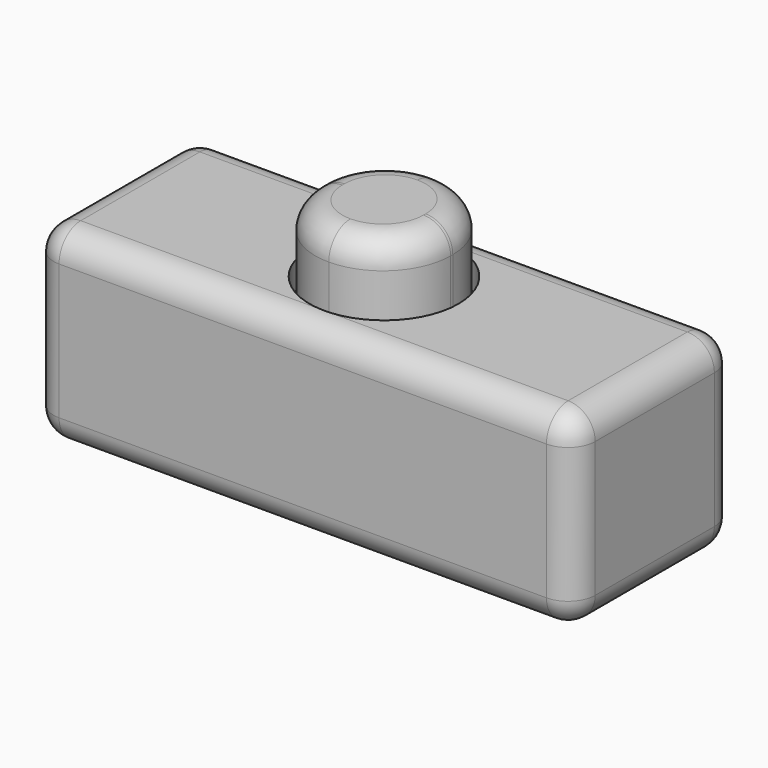
from build123d import *

# Parameters (mm, degrees)
F0_W     = 50.8
F0_H     = 19.05
F0_W_2   = 45.72
F0_H_2   = 13.97
F1_DEPTH = 12.7
F2_W     = 50.8
F2_H     = 19.05
F3_DEPTH = 2.54
F5_START = 0.508
F4_W     = 4.572
F4_H     = 2.794
F4_W_2   = 12.7
F4_H_2   = 5.08
F4_H_3   = 3.81
F5_DEPTH = 12.954
F6_R     = 6.34999
F7_W     = 50.8
F7_H     = 19.05
F7_R     = 6.985
F8_DEPTH = 2.54
F9_R     = 2.54
F10_R    = 2.54


# Not quite as in the source:
# - a fillet or chamfer is up to 0.001 mm smaller than in the source, because OpenCascade refuses the exact size


with BuildPart() as f1:
    # F0 (on Top) → F1 (new body)
    with BuildSketch(Plane.XY):
        Rectangle(F0_W, F0_H)
        Rectangle(F0_W_2, F0_H_2, mode=Mode.SUBTRACT)
    extrude(amount=F1_DEPTH)

    # F2 (on face) → F3 (join)
    with BuildSketch(Plane(origin=(0, 0, 0), x_dir=(1, 0, 0), z_dir=(0, 0, -1))):
        Rectangle(F2_W, F2_H)
    extrude(amount=F3_DEPTH)

    # F4 (on face) → F5 (join)
    with BuildSketch(Plane.XZ.offset(-6.985).offset(F5_START)):
        Polygon((-25.4, 0.254), (-25.4, -2.54), (20.828, -2.54), (20.828, 0.254), (-20.828, 0.254), align=None)
        with Locations((23.114, -1.143)):
            Rectangle(F4_W, F4_H)
        with BuildLine():
            Line((-20.828, 0.254), (20.828, 0.254))
            Line((20.828, 0.254), (20.828, 0.508))
            ThreePointArc((20.828, 0.508), (19.7166563034, 0.9891715443), (19.3070802744, 2.1288462099))
            Line((19.3070802744, 2.1288462099), (5.08, 7.62))
            Line((5.08, 7.62), (-5.08, 7.62))
            Line((-5.08, 7.62), (-19.3070802744, 2.1288462099))
            ThreePointArc((-19.3070802744, 2.1288462099), (-19.3047702633, 2.0804475914), (-19.304, 2.032))
            ThreePointArc((-19.304, 2.032), (-19.7503692655, 0.9543692655), (-20.828, 0.508))
            Line((-20.828, 0.508), (-20.828, 0.254))
        make_face()
        with BuildLine():
            ThreePointArc((19.3070802744, 2.1288462099), (19.7166563034, 0.9891715443), (20.828, 0.508))
            Line((20.828, 0.508), (20.828, 2.032))
            Line((20.828, 2.032), (19.558, 2.032))
            Line((19.558, 2.032), (19.3070802744, 2.1288462099))
        make_face()
        with BuildLine():
            Line((20.828, 2.032), (20.828, 0.508))
            ThreePointArc((20.828, 0.508), (21.9056307345, 0.9543692655), (22.352, 2.032))
            ThreePointArc((22.352, 2.032), (21.7251962822, 3.2639151071), (20.3603794867, 3.4824851104))
            Line((20.3603794867, 3.4824851104), (20.828, 3.302))
            Line((20.828, 3.302), (20.828, 2.032))
        make_face()
        with BuildLine():
            ThreePointArc((-20.3603794867, 3.4824851104), (-22.3335091013, 2.2686819509), (-20.828, 0.508))
            Line((-20.828, 0.508), (-20.828, 2.032))
            Line((-20.828, 2.032), (-20.828, 3.302))
            Line((-20.828, 3.302), (-20.3603794867, 3.4824851104))
        make_face()
        with BuildLine():
            Line((-20.828, 2.032), (-20.828, 0.508))
            ThreePointArc((-20.828, 0.508), (-19.7503692655, 0.9543692655), (-19.304, 2.032))
            ThreePointArc((-19.304, 2.032), (-19.3047702633, 2.0804475914), (-19.3070802744, 2.1288462099))
            Line((-19.3070802744, 2.1288462099), (-19.558, 2.032))
            Line((-19.558, 2.032), (-20.828, 2.032))
        make_face()
        with BuildLine():
            Line((19.558, 2.032), (20.828, 2.032))
            Line((20.828, 2.032), (20.828, 3.302))
            Line((20.828, 3.302), (20.3603794867, 3.4824851104))
            ThreePointArc((20.3603794867, 3.4824851104), (19.6252291828, 2.9679051027), (19.3070802744, 2.1288462099))
            Line((19.3070802744, 2.1288462099), (19.558, 2.032))
        make_face()
        with BuildLine():
            Line((5.08, 7.62), (19.3070802744, 2.1288462099))
            ThreePointArc((19.3070802744, 2.1288462099), (19.6252291828, 2.9679051027), (20.3603794867, 3.4824851104))
            Line((20.3603794867, 3.4824851104), (6.35, 8.89))
            Line((6.35, 8.89), (6.35, 7.62))
            Line((6.35, 7.62), (5.08, 7.62))
        make_face()
        with BuildLine():
            Line((-20.828, 3.302), (-20.828, 2.032))
            Line((-20.828, 2.032), (-19.558, 2.032))
            Line((-19.558, 2.032), (-19.3070802744, 2.1288462099))
            ThreePointArc((-19.3070802744, 2.1288462099), (-19.6252291828, 2.9679051027), (-20.3603794867, 3.4824851104))
            Line((-20.3603794867, 3.4824851104), (-20.828, 3.302))
        make_face()
        with BuildLine():
            Line((-6.35, 8.89), (-20.3603794867, 3.4824851104))
            ThreePointArc((-20.3603794867, 3.4824851104), (-19.6252291828, 2.9679051027), (-19.3070802744, 2.1288462099))
            Line((-19.3070802744, 2.1288462099), (-5.08, 7.62))
            Line((-5.08, 7.62), (-6.35, 7.62))
            Line((-6.35, 7.62), (-6.35, 8.89))
        make_face()
        Polygon((-5.08, 7.62), (5.08, 7.62), (6.35, 7.62), (6.35, 8.89), (6.35, 12.7), (-6.35, 12.7), (-6.35, 8.89), (-6.35, 7.62), align=None)
        with Locations((0, 15.24)):
            Rectangle(F4_W_2, F4_H_2)
        with Locations((0, 19.685)):
            Rectangle(F4_W_2, F4_H_3)
    extrude(amount=F5_DEPTH)

    # F6 (radius 6.35 in the source; OpenCascade refuses exactly that, so slightly less here)
    f6_edges = [f1.edges().sort_by_distance(p)[0] for p in [
        (-6.35, -6.477, 15.24),
        (6.35, -6.477, 15.24),
        (6.35, 6.477, 15.24),
        (-6.35, 6.477, 15.24),
    ]]
    fillet(f6_edges, radius=F6_R)

    # F7 (on face) → F8 (join)
    with BuildSketch(Plane.XY.offset(12.7)):
        Rectangle(F7_W, F7_H)
        Circle(F7_R, mode=Mode.SUBTRACT)
    extrude(amount=F8_DEPTH)

    # F9
    f9_edges = [f1.edges().sort_by_distance(p)[0] for p in [
        (-25.4, 9.525, 6.35),
        (-25.4, 0, 15.24),
        (-25.4, -9.525, 6.35),
        (-25.4, 0, -2.54),
        (25.4, 9.525, 6.35),
        (25.4, 0, -2.54),
        (25.4, -9.525, 6.35),
        (25.4, 0, 15.24),
        (0, -9.525, 15.24),
        (0, -9.525, -2.54),
        (0, 9.525, -2.54),
        (0, 9.525, 15.24),
    ]]
    fillet(f9_edges, radius=F9_R)

    # F10
    f10_edges = [f1.edges().sort_by_distance(p)[0] for p in [
        (4.490131, -4.617131, 21.59),
    ]]
    fillet(f10_edges, radius=F10_R)


solid = f1.part
